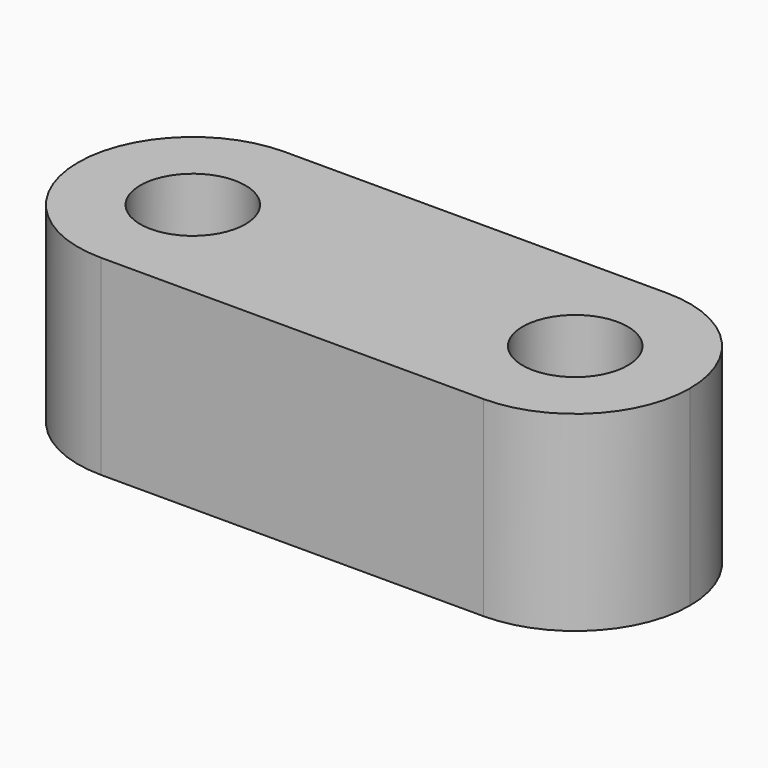
from build123d import *

# Parameters (mm, degrees)
F0_W     = 32
F0_H     = 12
F0_R     = 2.75
F1_DEPTH = 10
F2_R     = 5.99999


# Not quite as in the source:
# - a fillet or chamfer is up to 0.001 mm smaller than in the source, because OpenCascade refuses the exact size


with BuildPart() as f1:
    # F0 (on Top) → F1 (new body)
    with BuildSketch(Plane.XY):
        with Locations((10, 0)):
            Rectangle(F0_W, F0_H)
        Circle(F0_R, mode=Mode.SUBTRACT)
        with Locations((20, 0)):
            Circle(F0_R, mode=Mode.SUBTRACT)
    extrude(amount=F1_DEPTH)

    # F2 (radius 6 in the source; OpenCascade refuses exactly that, so slightly less here)
    f2_edges = [f1.edges().sort_by_distance(p)[0] for p in [
        (-6, -6, 5),
        (-6, 6, 5),
        (26, -6, 5),
        (26, 6, 5),
    ]]
    fillet(f2_edges, radius=F2_R)


solid = f1.part
